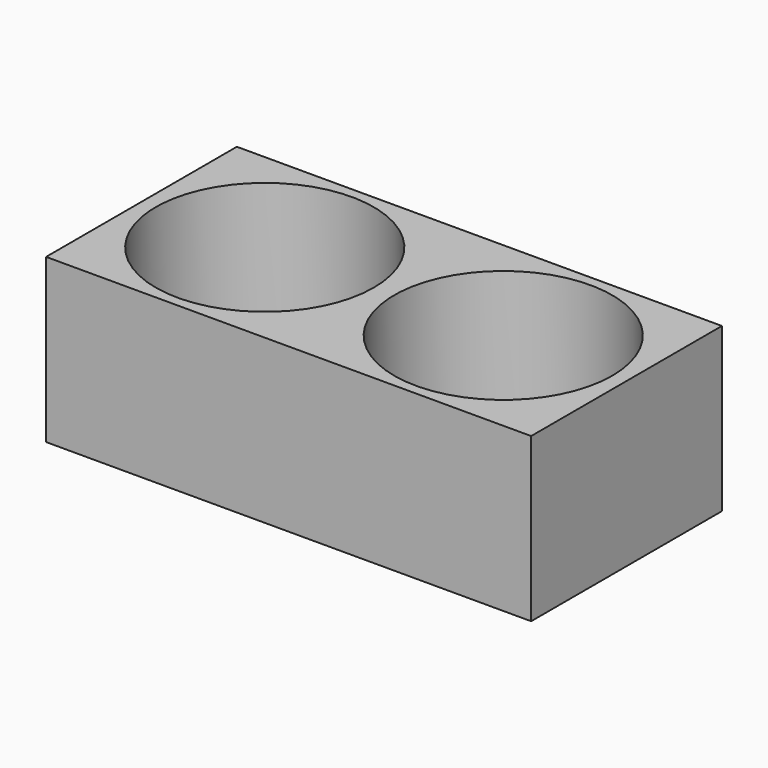
from build123d import *

# Parameters (mm, degrees)
F2_W     = 23.8
F2_H     = 11.7
F3_DEPTH = 8
F4_R     = 5.35
F5_DEPTH = 6


# Not quite as in the source:
# - a feature names something its author has since deleted; it is built from what else it names


with BuildPart() as f3:
    # F2 (on Top) → F3 (new body)
    with BuildSketch(Plane.XY):
        Rectangle(F2_W, F2_H)
    extrude(amount=F3_DEPTH)

    # F4 (on face) → F5 (cut)
    with BuildSketch(Plane.XY.offset(8)):
        with Locations((-5.85, 0)):
            Circle(F4_R)
        with Locations((5.85, 0)):
            Circle(F4_R)
    extrude(amount=-F5_DEPTH, mode=Mode.SUBTRACT)


solid = f3.part
